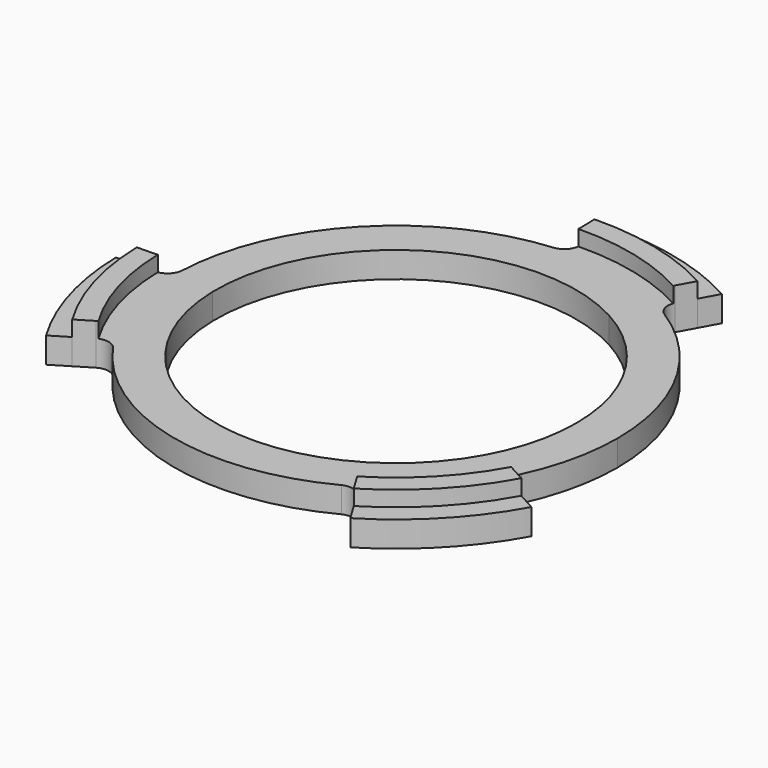
from build123d import *

# Parameters (mm, degrees)
F1_DEPTH     = 4
F2_DEPTH     = 2.5
F3_T3_DEPTH  = 2.5
F3_T6_DEPTH  = 6.1298487604
F3_S8_R      = 22.75
F3_T9_DEPTH  = 5
F3_T12_DEPTH = 2.5
F3_T15_DEPTH = 6.1298487604
F3_S16_R     = 22.75
F3_T17_DEPTH = 5
F3_T21_DEPTH = 2.5
F3_T24_DEPTH = 6.1298487604
F3_S25_R     = 22.75
F3_T26_DEPTH = 5
F3_T30_DEPTH = 2.5
F3_T33_DEPTH = 6.1298487604
F3_S35_R     = 22.75
F3_T36_DEPTH = 5
F3_T39_DEPTH = 2.5
F3_T42_DEPTH = 6.1298487604
F3_S44_R     = 22.75
F3_T45_DEPTH = 5
F3_T48_DEPTH = 2.5
F3_T51_DEPTH = 6.1298487604
F3_S53_R     = 22.75
F3_T54_DEPTH = 5


# Not quite as in the source:
# - a fillet or chamfer that OpenCascade refuses, or shapes differently, is made with other operations: its cross-section is extruded or revolved along the edge and cut away or added


with BuildPart() as f1:
    # F0 (on Top) → F1 (new body)
    with BuildSketch(Plane.XY):
        with BuildLine():
            Line((10.952278028, 19.9401631387), (11.9151156568, 21.6931445135))
            ThreePointArc((11.9151156568, 21.6931445135), (5.8945189879, 24.0378273956), (-0.5277794089, 24.7443720651))
            Line((-0.5277794089, 24.7443720651), (-0.4851305678, 22.7448268477))
            ThreePointArc((-0.4851305678, 22.7448268477), (5.4181942212, 22.095376697), (10.952278028, 19.9401631387))
        make_face()
    extrude(amount=F1_DEPTH)



with BuildPart() as f1b:
    # F0 (on Top) → F1, piece 2 (new body)
    with BuildSketch(Plane.XY):
        with BuildLine():
            Line((-22.7448268477, -0.4851305678), (-24.7443720651, -0.5277794089))
            ThreePointArc((-24.7443720651, -0.5277794089), (-23.7646286703, -6.9141105112), (-21.1653651046, -12.8292564083))
            Line((-21.1653651046, -12.8292564083), (-19.4550325709, -11.7925488197))
            ThreePointArc((-19.4550325709, -11.7925488197), (-21.8442546364, -6.3553945103), (-22.7448268477, -0.4851305678))
        make_face()
    extrude(amount=F1_DEPTH)


with BuildPart() as f1c:
    # F0 (on Top) → F1, piece 3 (new body)
    with BuildSketch(Plane.XY):
        with BuildLine():
            ThreePointArc((12.8292564083, -21.1653651046), (17.8701096825, -17.1237168844), (21.6931445135, -11.9151156568))
            Line((21.6931445135, -11.9151156568), (19.9401631387, -10.952278028))
            ThreePointArc((19.9401631387, -10.952278028), (16.4260604152, -15.7399821867), (11.7925488197, -19.4550325709))
            Line((11.7925488197, -19.4550325709), (12.8292564083, -21.1653651046))
        make_face()
    extrude(amount=F1_DEPTH)


with BuildPart() as f1_1:
    add(f1.part)

    add(f1b.part)  # F2 merges F1b

    add(f1c.part)  # F2 merges F1c
    # F0 (on Top) → F2 (join)
    with BuildSketch(Plane.XY):
        with BuildLine():
            Line((11.9151156568, 21.6931445135), (12.8779532856, 23.4461258884))
            ThreePointArc((12.8779532856, 23.4461258884), (6.3708437546, 25.9802780943), (-0.5704282501, 26.7439172825))
            Line((-0.5704282501, 26.7439172825), (-0.5277794089, 24.7443720651))
            ThreePointArc((-0.5277794089, 24.7443720651), (5.8945189879, 24.0378273956), (11.9151156568, 21.6931445135))
        make_face()
        with BuildLine():
            Line((-24.7443720651, -0.5277794089), (-26.7439172825, -0.5704282501))
            ThreePointArc((-26.7439172825, -0.5704282501), (-25.6850027043, -7.4728265121), (-22.8756976383, -13.8659639968))
            Line((-22.8756976383, -13.8659639968), (-21.1653651046, -12.8292564083))
            ThreePointArc((-21.1653651046, -12.8292564083), (-23.7646286703, -6.9141105112), (-24.7443720651, -0.5277794089))
        make_face()
        with BuildLine():
            ThreePointArc((13.8659639968, -22.8756976383), (19.3141589497, -18.5074515821), (23.4461258884, -12.8779532856))
            Line((23.4461258884, -12.8779532856), (21.6931445135, -11.9151156568))
            ThreePointArc((21.6931445135, -11.9151156568), (17.8701096825, -17.1237168844), (12.8292564083, -21.1653651046))
            Line((12.8292564083, -21.1653651046), (13.8659639968, -22.8756976383))
        make_face()
        with BuildLine():
            Line((8.4248292523, 15.3385870298), (10.35050451, 18.8445497794))
            ThreePointArc((10.35050451, 18.8445497794), (5.120491242, 20.8813450103), (-0.4584750421, 21.4951110868))
            Line((-0.4584750421, 21.4951110868), (-0.3731773599, 17.4960206521))
            ThreePointArc((-0.3731773599, 17.4960206521), (4.1678417086, 16.9964436131), (8.4248292523, 15.3385870298))
        make_face()
        with BuildLine():
            Line((-0.3731773599, 17.4960206521), (-0.4584750421, 21.4951110868))
            ThreePointArc((-0.4584750421, 21.4951110868), (-15.5235296231, 14.8751480006), (-21.4951110868, -0.4584750421))
            Line((-21.4951110868, -0.4584750421), (-17.4960206521, -0.3731773599))
            ThreePointArc((-17.4960206521, -0.3731773599), (-12.6354310886, 12.1076786051), (-0.3731773599, 17.4960206521))
        make_face()
        with BuildLine():
            Line((-17.4960206521, -0.3731773599), (-21.4951110868, -0.4584750421))
            ThreePointArc((-21.4951110868, -0.4584750421), (-20.6440208651, -6.0061970097), (-18.3860747373, -11.1446065769))
            Line((-18.3860747373, -11.1446065769), (-14.9654096699, -9.0711913998))
            ThreePointArc((-14.9654096699, -9.0711913998), (-16.8032727972, -4.8887650079), (-17.4960206521, -0.3731773599))
        make_face()
        with BuildLine():
            ThreePointArc((-18.3860747373, -11.1446065769), (-5.120491242, -20.8813450103), (11.1446065769, -18.3860747373))
            Line((11.1446065769, -18.3860747373), (9.0711913998, -14.9654096699))
            ThreePointArc((9.0711913998, -14.9654096699), (-4.1678417086, -16.9964436131), (-14.9654096699, -9.0711913998))
            Line((-14.9654096699, -9.0711913998), (-18.3860747373, -11.1446065769))
        make_face()
        with BuildLine():
            ThreePointArc((11.1446065769, -18.3860747373), (15.5235296231, -14.8751480006), (18.8445497794, -10.35050451))
            Line((18.8445497794, -10.35050451), (15.3385870298, -8.4248292523))
            ThreePointArc((15.3385870298, -8.4248292523), (12.6354310886, -12.1076786051), (9.0711913998, -14.9654096699))
            Line((9.0711913998, -14.9654096699), (11.1446065769, -18.3860747373))
        make_face()
        with BuildLine():
            ThreePointArc((21.5, 0), (18.5038623936, 10.9479256719), (10.35050451, 18.8445497794))
            Line((10.35050451, 18.8445497794), (8.4248292523, 15.3385870298))
            ThreePointArc((8.4248292523, 15.3385870298), (15.0612833436, 8.9111022911), (17.5, 0))
            ThreePointArc((17.5, 0), (16.9510364435, -4.3488347278), (15.3385870298, -8.4248292523))
            Line((15.3385870298, -8.4248292523), (18.8445497794, -10.35050451))
            ThreePointArc((18.8445497794, -10.35050451), (20.8255590592, -5.3428540941), (21.5, 0))
        make_face()
        with BuildLine():
            Line((-21.4951110868, -0.4584750421), (-22.7448268477, -0.4851305678))
            ThreePointArc((-22.7448268477, -0.4851305678), (-21.8442546364, -6.3553945103), (-19.4550325709, -11.7925488197))
            Line((-19.4550325709, -11.7925488197), (-18.3860747373, -11.1446065769))
            ThreePointArc((-18.3860747373, -11.1446065769), (-20.6440208651, -6.0061970097), (-21.4951110868, -0.4584750421))
        make_face()
        with BuildLine():
            ThreePointArc((11.7925488197, -19.4550325709), (16.4260604152, -15.7399821867), (19.9401631387, -10.952278028))
            Line((19.9401631387, -10.952278028), (18.8445497794, -10.35050451))
            ThreePointArc((18.8445497794, -10.35050451), (15.5235296231, -14.8751480006), (11.1446065769, -18.3860747373))
            Line((11.1446065769, -18.3860747373), (11.7925488197, -19.4550325709))
        make_face()
        with BuildLine():
            Line((10.35050451, 18.8445497794), (10.952278028, 19.9401631387))
            ThreePointArc((10.952278028, 19.9401631387), (5.4181942212, 22.095376697), (-0.4851305678, 22.7448268477))
            Line((-0.4851305678, 22.7448268477), (-0.4584750421, 21.4951110868))
            ThreePointArc((-0.4584750421, 21.4951110868), (5.120491242, 20.8813450103), (10.35050451, 18.8445497794))
        make_face()
    extrude(amount=F2_DEPTH)

    # F3: fillet of radius 1.5 on 6 edges, made by hand


with BuildPart() as f3_tool1:
    # F3_s2 → F3_t3 (new body)
    with BuildSketch(Plane.XY):
        with BuildLine():
            ThreePointArc((-19.6279317172, -11.8968828329), (-18.539917703, -11.7117398386), (-17.6192977153, -12.3204362009))
            Line((-17.6192977153, -12.3204362009), (-17.496258175, -12.2343998089))
            ThreePointArc((-17.496258175, -12.2343998089), (-17.8866718738, -11.6569137348), (-18.2576830085, -11.0667827169))
            Line((-18.2576830085, -11.0667827169), (-18.4638985973, -11.016214848))
            ThreePointArc((-18.4638985973, -11.016214848), (-19.0847234165, -11.3925240093), (-19.7057555772, -11.768491104))
            Line((-19.7057555772, -11.768491104), (-19.6279317172, -11.8968828329))
        make_face()
    extrude(amount=F3_T3_DEPTH)


with BuildPart() as f3_tool4:
    # F3_s5 → F3_t6 (new body)
    with BuildSketch(Plane.XY):
        with BuildLine():
            ThreePointArc((-19.6279317172, -11.8968828329), (-18.539917703, -11.7117398386), (-17.6192977153, -12.3204362009))
            Line((-17.6192977153, -12.3204362009), (-17.496258175, -12.2343998089))
            ThreePointArc((-17.496258175, -12.2343998089), (-17.8866718738, -11.6569137348), (-18.2576830085, -11.0667827169))
            Line((-18.2576830085, -11.0667827169), (-18.4638985973, -11.016214848))
            ThreePointArc((-18.4638985973, -11.016214848), (-19.0847234165, -11.3925240093), (-19.7057555772, -11.768491104))
            Line((-19.7057555772, -11.768491104), (-19.6279317172, -11.8968828329))
        make_face()
    extrude(amount=F3_T6_DEPTH)

    split(bisect_by=Plane.XY.offset(4), keep=Keep.BOTTOM)

    # F3_s8 → F3_t9 (cut, symmetric)
    with BuildSketch(Plane.XY.offset(3.1)):
        Circle(F3_S8_R)
    extrude(amount=F3_T9_DEPTH, both=True, mode=Mode.SUBTRACT)


with BuildPart() as f3_tool10:
    # F3_s11 → F3_t12 (new body)
    with BuildSketch(Plane.XY):
        with BuildLine():
            ThreePointArc((11.8975669659, -19.6275170342), (11.0186307447, -18.9600415346), (9.9208540079, -19.0737897628))
            Line((9.9208540079, -19.0737897628), (9.851574441, -18.9405931757))
            ThreePointArc((9.851574441, -18.9405931757), (10.4648544282, -18.6092313204), (11.0667827169, -18.2576830085))
            Line((11.0667827169, -18.2576830085), (11.2729983057, -18.3082508774))
            ThreePointArc((11.2729983057, -18.3082508774), (11.649307467, -18.9290756965), (12.0259586947, -19.5496931742))
            Line((12.0259586947, -19.5496931742), (11.8975669659, -19.6275170342))
        make_face()
    extrude(amount=F3_T12_DEPTH)


with BuildPart() as f3_tool13:
    # F3_s14 → F3_t15 (new body)
    with BuildSketch(Plane.XY):
        with BuildLine():
            ThreePointArc((11.8975669659, -19.6275170342), (11.0186307447, -18.9600415346), (9.9208540079, -19.0737897628))
            Line((9.9208540079, -19.0737897628), (9.851574441, -18.9405931757))
            ThreePointArc((9.851574441, -18.9405931757), (10.4648544282, -18.6092313204), (11.0667827169, -18.2576830085))
            Line((11.0667827169, -18.2576830085), (11.2729983057, -18.3082508774))
            ThreePointArc((11.2729983057, -18.3082508774), (11.649307467, -18.9290756965), (12.0259586947, -19.5496931742))
            Line((12.0259586947, -19.5496931742), (11.8975669659, -19.6275170342))
        make_face()
    extrude(amount=F3_T15_DEPTH)

    # F3_s16 → F3_t17 (cut, symmetric)
    with BuildSketch(Plane.XY.offset(3.1)):
        Circle(F3_S16_R)
    extrude(amount=F3_T17_DEPTH, both=True, mode=Mode.SUBTRACT)

    split(bisect_by=Plane.XY.offset(4), keep=Keep.BOTTOM)


with BuildPart() as f3_tool19:
    # F3_s20 → F3_t21 (new body)
    with BuildSketch(Plane.XY):
        with BuildLine():
            ThreePointArc((19.4794595933, -9.0985413178), (19.4126230743, -10.2001697956), (20.1169686177, -11.0498460744))
            Line((20.1169686177, -11.0498460744), (20.0446900489, -11.1814393786))
            ThreePointArc((20.0446900489, -11.1814393786), (19.4085769135, -10.8315932982), (18.7722712106, -10.4820978141))
            Line((18.7722712106, -10.4820978141), (18.7129564753, -10.2782259411))
            ThreePointArc((18.7129564753, -10.2782259411), (19.038519361, -9.6618553644), (19.3434301221, -9.0350041463))
            Line((19.3434301221, -9.0350041463), (19.4794595933, -9.0985413178))
        make_face()
    extrude(amount=F3_T21_DEPTH)


with BuildPart() as f3_tool22:
    # F3_s23 → F3_t24 (new body)
    with BuildSketch(Plane.XY):
        with BuildLine():
            ThreePointArc((19.4794595933, -9.0985413178), (19.4126230743, -10.2001697956), (20.1169686177, -11.0498460744))
            Line((20.1169686177, -11.0498460744), (20.0446900489, -11.1814393786))
            ThreePointArc((20.0446900489, -11.1814393786), (19.4085769135, -10.8315932982), (18.7722712106, -10.4820978141))
            Line((18.7722712106, -10.4820978141), (18.7129564753, -10.2782259411))
            ThreePointArc((18.7129564753, -10.2782259411), (19.038519361, -9.6618553644), (19.3434301221, -9.0350041463))
            Line((19.3434301221, -9.0350041463), (19.4794595933, -9.0985413178))
        make_face()
    extrude(amount=F3_T24_DEPTH)

    # F3_s25 → F3_t26 (cut, symmetric)
    with BuildSketch(Plane.XY.offset(3.1)):
        Circle(F3_S25_R)
    extrude(amount=F3_T26_DEPTH, both=True, mode=Mode.SUBTRACT)

    split(bisect_by=Plane.XY.offset(4), keep=Keep.BOTTOM)


with BuildPart() as f3_tool28:
    # F3_s29 → F3_t30 (new body)
    with BuildSketch(Plane.XY):
        with BuildLine():
            ThreePointArc((11.0491448819, 20.1173537527), (10.9105622534, 19.0224349072), (11.557959477, 18.1286064795))
            Line((11.557959477, 18.1286064795), (11.4772476324, 18.002010321))
            ThreePointArc((11.4772476324, 18.002010321), (10.8836398543, 18.367445442), (10.2782259411, 18.7129564753))
            Line((10.2782259411, 18.7129564753), (10.2189112058, 18.9168283483))
            ThreePointArc((10.2189112058, 18.9168283483), (10.5684066899, 19.5531340512), (10.9175515777, 20.1896323216))
            Line((10.9175515777, 20.1896323216), (11.0491448819, 20.1173537527))
        make_face()
    extrude(amount=F3_T30_DEPTH)


with BuildPart() as f3_tool31:
    # F3_s32 → F3_t33 (new body)
    with BuildSketch(Plane.XY):
        with BuildLine():
            ThreePointArc((11.0491448819, 20.1173537527), (10.9105622534, 19.0224349072), (11.557959477, 18.1286064795))
            Line((11.557959477, 18.1286064795), (11.4772476324, 18.002010321))
            ThreePointArc((11.4772476324, 18.002010321), (10.8836398543, 18.367445442), (10.2782259411, 18.7129564753))
            Line((10.2782259411, 18.7129564753), (10.2189112058, 18.9168283483))
            ThreePointArc((10.2189112058, 18.9168283483), (10.5684066899, 19.5531340512), (10.9175515777, 20.1896323216))
            Line((10.9175515777, 20.1896323216), (11.0491448819, 20.1173537527))
        make_face()
    extrude(amount=F3_T33_DEPTH)

    split(bisect_by=Plane.XY.offset(4), keep=Keep.BOTTOM)

    # F3_s35 → F3_t36 (cut, symmetric)
    with BuildSketch(Plane.XY.offset(3.1)):
        Circle(F3_S35_R)
    extrude(amount=F3_T36_DEPTH, both=True, mode=Mode.SUBTRACT)


with BuildPart() as f3_tool37:
    # F3_s38 → F3_t39 (new body)
    with BuildSketch(Plane.XY):
        with BuildLine():
            ThreePointArc((-1.8601618781, 21.4189775187), (-0.8727053713, 21.9119096342), (-0.4890369005, 22.9467289073))
            Line((-0.4890369005, 22.9467289073), (-0.3389344717, 22.9499304826))
            ThreePointArc((-0.3389344717, 22.9499304826), (-0.323853497, 22.2241173075), (-0.3083726133, 21.4983126622))
            Line((-0.3083726133, 21.4983126622), (-0.4552734668, 21.3450086581))
            ThreePointArc((-0.4552734668, 21.3450086581), (-1.1518474872, 21.3187690993), (-1.847171947, 21.2694039552))
            Line((-1.847171947, 21.2694039552), (-1.8601618781, 21.4189775187))
        make_face()
    extrude(amount=F3_T39_DEPTH)


with BuildPart() as f3_tool40:
    # F3_s41 → F3_t42 (new body)
    with BuildSketch(Plane.XY):
        with BuildLine():
            ThreePointArc((-1.8601618781, 21.4189775187), (-0.8727053713, 21.9119096342), (-0.4890369005, 22.9467289073))
            Line((-0.4890369005, 22.9467289073), (-0.3389344717, 22.9499304826))
            ThreePointArc((-0.3389344717, 22.9499304826), (-0.323853497, 22.2241173075), (-0.3083726133, 21.4983126622))
            Line((-0.3083726133, 21.4983126622), (-0.4552734668, 21.3450086581))
            ThreePointArc((-0.4552734668, 21.3450086581), (-1.1518474872, 21.3187690993), (-1.847171947, 21.2694039552))
            Line((-1.847171947, 21.2694039552), (-1.8601618781, 21.4189775187))
        make_face()
    extrude(amount=F3_T42_DEPTH)

    split(bisect_by=Plane.XY.offset(4), keep=Keep.BOTTOM)

    # F3_s44 → F3_t45 (cut, symmetric)
    with BuildSketch(Plane.XY.offset(3.1)):
        Circle(F3_S44_R)
    extrude(amount=F3_T45_DEPTH, both=True, mode=Mode.SUBTRACT)


with BuildPart() as f3_tool46:
    # F3_s47 → F3_t48 (new body)
    with BuildSketch(Plane.XY):
        with BuildLine():
            ThreePointArc((-21.4788134849, 0.9451832833), (-21.9291929982, -0.0623933726), (-22.9467118477, -0.4898367186))
            Line((-22.9467118477, -0.4898367186), (-22.9435102724, -0.6399391474))
            ThreePointArc((-22.9435102724, -0.6399391474), (-22.2177141568, -0.6240583546), (-21.4919095115, -0.6085774709))
            Line((-21.4919095115, -0.6085774709), (-21.3450086581, -0.4552734668))
            ThreePointArc((-21.3450086581, -0.4552734668), (-21.3484942825, 0.2417858785), (-21.3288220733, 0.9385828547))
            Line((-21.3288220733, 0.9385828547), (-21.4788134849, 0.9451832833))
        make_face()
    extrude(amount=F3_T48_DEPTH)


with BuildPart() as f3_tool49:
    # F3_s50 → F3_t51 (new body)
    with BuildSketch(Plane.XY):
        with BuildLine():
            ThreePointArc((-21.4788134849, 0.9451832833), (-21.9291929982, -0.0623933726), (-22.9467118477, -0.4898367186))
            Line((-22.9467118477, -0.4898367186), (-22.9435102724, -0.6399391474))
            ThreePointArc((-22.9435102724, -0.6399391474), (-22.2177141568, -0.6240583546), (-21.4919095115, -0.6085774709))
            Line((-21.4919095115, -0.6085774709), (-21.3450086581, -0.4552734668))
            ThreePointArc((-21.3450086581, -0.4552734668), (-21.3484942825, 0.2417858785), (-21.3288220733, 0.9385828547))
            Line((-21.3288220733, 0.9385828547), (-21.4788134849, 0.9451832833))
        make_face()
    extrude(amount=F3_T51_DEPTH)

    split(bisect_by=Plane.XY.offset(4), keep=Keep.BOTTOM)

    # F3_s53 → F3_t54 (cut, symmetric)
    with BuildSketch(Plane.XY.offset(3.1)):
        Circle(F3_S53_R)
    extrude(amount=F3_T54_DEPTH, both=True, mode=Mode.SUBTRACT)


with BuildPart() as f1_2:
    add(f1_1.part)

    # F3_t55: union F3_tool1, F3_tool4, F3_tool10, F3_tool13, F3_tool19, F3_tool22, F3_tool28, F3_tool31, F3_tool37, F3_tool40, F3_tool46, F3_tool49
    add([f3_tool1.part, f3_tool4.part, f3_tool10.part, f3_tool13.part, f3_tool19.part, f3_tool22.part, f3_tool28.part, f3_tool31.part, f3_tool37.part, f3_tool40.part, f3_tool46.part, f3_tool49.part])


solid = f1_2.part
